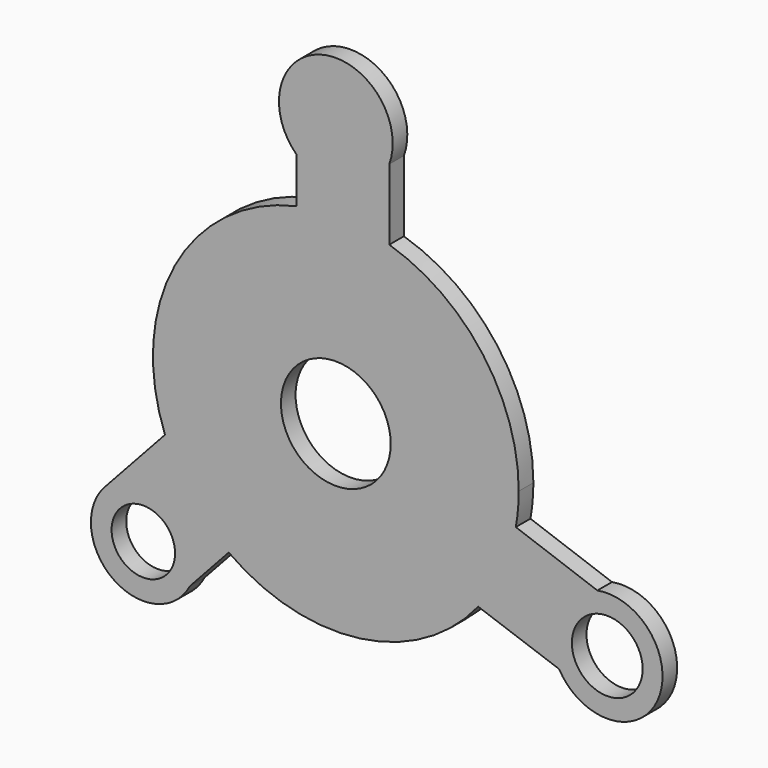
from build123d import *

# Parameters (mm, degrees)
F0_R     = 6
F3_DEPTH = 2
F4_R     = 2.937220037
F4_R_2   = 2.9600798579
F4_R_3   = 3.1369542822
F5_DEPTH = 25
F6_R     = 3.870285665
F6_R_2   = 3.4699614842
F7_DEPTH = 3


# Not quite as in the source:
# - the program builds the solid bodies; features that only make, move or delete a surface that nothing else refers to are left out


with BuildPart() as f3:
    # F0 (on Front) → F3 (new body)
    with BuildSketch(Plane.XZ):
        with BuildLine():
            ThreePointArc((19.6806687258, 19.8017779916), (19.9200072103, 21.5744676649), (20, 23.3614519238))
            ThreePointArc((20, 23.3614519238), (16.0767393697, 35.2584452936), (5.8461548761, 42.4879380926))
            ThreePointArc((5.8461548761, 42.4879380926), (0.7853649586, 43.3460260219), (-4.327156771, 42.8877345777))
            ThreePointArc((-4.327156771, 42.8877345777), (-17.6128349493, 32.8371073128), (-18.6785365647, 16.2121672183))
            ThreePointArc((-18.6785365647, 16.2121672183), (-15.8565738824, 11.1725608869), (-11.7121291204, 7.1495417506))
            ThreePointArc((-11.7121291204, 7.1495417506), (2.6572751847, 3.5387657135), (15.5683835849, 10.8065551679))
            ThreePointArc((15.5683835849, 10.8065551679), (18.189349373, 15.0459501719), (19.6806687258, 19.8017779916))
        make_face()
        with Locations((0, 23.3614519238)):
            Circle(F0_R, mode=Mode.SUBTRACT)
        with BuildLine():
            ThreePointArc((-4.327156771, 42.8877345777), (0.7853649586, 43.3460260219), (5.8461548761, 42.4879380926))
            Line((5.8461548761, 42.4879380926), (5.8461548761, 50.2402076719))
            ThreePointArc((5.8461548761, 50.2402076719), (-1.3985114704, 58.4135951865), (-4.327156771, 47.891594871))
            Line((-4.327156771, 47.891594871), (-4.327156771, 42.8877345777))
        make_face()
        with BuildLine():
            Line((28.5979291758, 16.5996841985), (19.6806687258, 19.8017779916))
            ThreePointArc((19.6806687258, 19.8017779916), (18.189349373, 15.0459501719), (15.5683835849, 10.8065551679))
            Line((15.5683835849, 10.8065551679), (24.4160998295, 7.6740266873))
            ThreePointArc((24.4160998295, 7.6740266873), (35.1512386763, 8.0868826224), (28.5979291758, 16.5996841985))
        make_face()
        with BuildLine():
            ThreePointArc((-11.7121291204, 7.1495417506), (-15.8565738824, 11.1725608869), (-18.6785365647, 16.2121672183))
            Line((-18.6785365647, 16.2121672183), (-25.2698698947, 9.0414457989))
            ThreePointArc((-25.2698698947, 9.0414457989), (-24.3393468403, 0.4704595262), (-15.965672237, 2.5221058119))
            Line((-15.965672237, 2.5221058119), (-11.7121291204, 7.1495417506))
        make_face()
    extrude(amount=F3_DEPTH)

    # F4 (on Front) → F5 (cut)
    with BuildSketch(Plane.XZ):
        with Locations((0, 53.6376424134)):
            Circle(F4_R)
        with Locations((29.5011680573, 10.3136152029)):
            Circle(F4_R_2)
        with Locations((-20.7987613976, 4.8063262366)):
            Circle(F4_R_3)
    extrude(amount=-F5_DEPTH, mode=Mode.SUBTRACT)

    # F6 (on face) → F7 (cut)
    with BuildSketch(Plane.XZ.offset(2)):
        with Locations((29.6770948917, 10.6516163796)):
            Circle(F6_R)
        with Locations((-21.0510119796, 5.1634679548)):
            Circle(F6_R_2)
    extrude(amount=-F7_DEPTH, mode=Mode.SUBTRACT)


solid = f3.part
